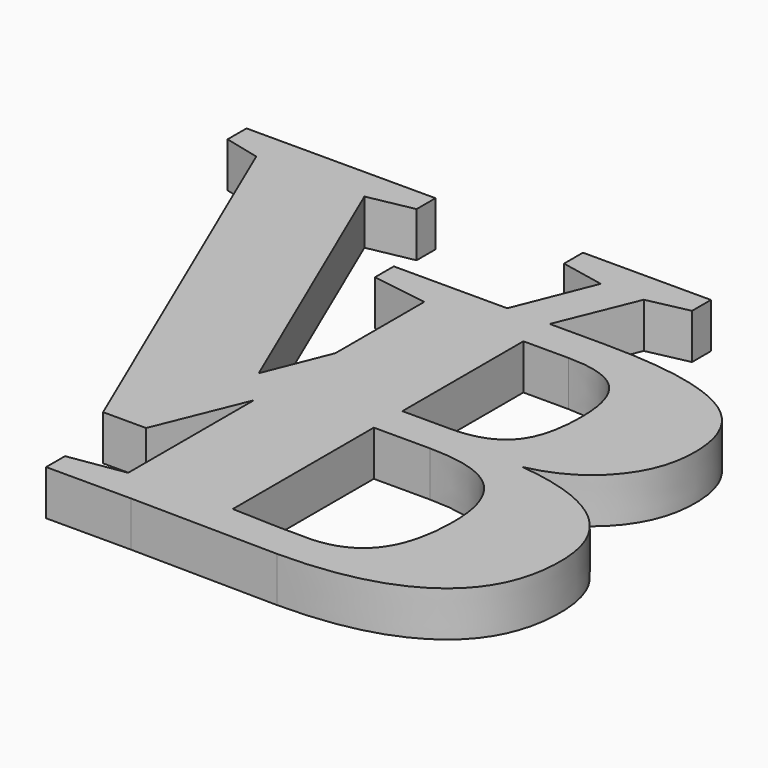
from build123d import *

# Parameters (mm, degrees)
F0_TEXT_SIZE = 56.0850293065
F1_DEPTH     = 3.81
F2_TEXT_SIZE = 56.0850293065
F3_DEPTH     = 3.81


# Not quite as in the source:
# - Text() gives the source's letters only with a copy of the font that has no kerning and outlines rounded to 1/6400 em; it was checked with that copy


with BuildPart() as f1:
    # F0 (on Top) → F1 (new body)
    with BuildSketch(Plane.XY):
        with Locations((-29.9723986536, -20.1932229102)):
            Text('V', F0_TEXT_SIZE, font='Tinos', font_style=FontStyle.BOLD, text_align=(TextAlign.LEFT, TextAlign.BOTTOM))
    extrude(amount=F1_DEPTH)

    # F2 (on Top) → F3 (join)
    with BuildSketch(Plane.XY):
        with Locations((-10.3640798479, -29.5209521428)):
            Text('B', F2_TEXT_SIZE, font='Tinos', font_style=FontStyle.BOLD, text_align=(TextAlign.LEFT, TextAlign.BOTTOM))
    extrude(amount=F3_DEPTH)


solid = f1.part
